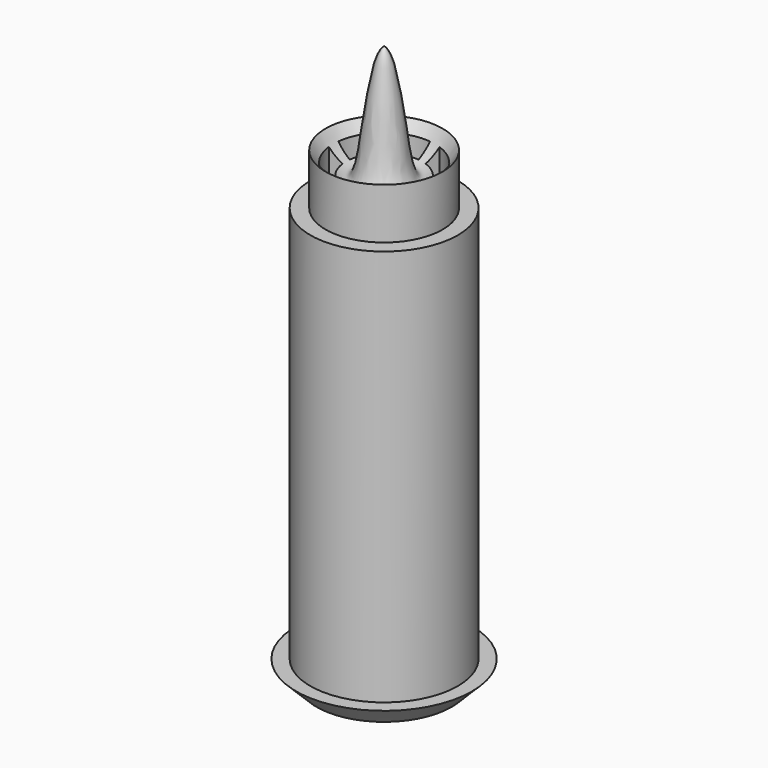
from build123d import *

# Parameters (mm, degrees)
F2_SIZE2  = 1.99999
F2_SIZE   = 1.99999
F5_R      = 5.75
F6_DEPTH  = 25
F7_R      = 5.75
F8_DEPTH  = 25
F10_DEPTH = 25


# Not quite as in the source:
# - a fillet or chamfer is up to 0.001 mm smaller than in the source, because OpenCascade refuses the exact size


with BuildPart() as f1:
    # F0 (on Front) → F1 (revolve)
    with BuildSketch(Plane.XZ):
        with BuildLine():
            Line((8.64674, 2), (7.25, 2))
            Line((7.25, 2), (7.25, 41))
            Line((7.25, 41), (5.75, 41))
            Line((5.75, 41), (5.75, 40))
            Line((5.75, 40), (4.75, 40))
            Line((4.75, 40), (4.75, 39))
            ThreePointArc((4.75, 39), (5.4571067812, 38.7071067812), (5.75, 38))
            Line((5.75, 38), (5.75, 4.9999998882))
            ThreePointArc((5.75, 4.9999998882), (5.4571067812, 4.2928931071), (4.75, 3.9999998882))
            Line((4.75, 3.9999998882), (4.75, 2.9999998882))
            Line((4.75, 2.9999998882), (5.75, 2.9999998882))
            Line((5.75, 2.9999998882), (5.75, 0))
            Line((5.75, 0), (8.64674, 0))
            Line((8.64674, 0), (8.64674, 2))
        make_face()
    revolve(axis=Axis((0, 0, 27.7979653329), (0, 0, 1)))

    # F2 (size 2 and 2 in the source; OpenCascade refuses exactly that, so slightly less here)
    f2_edges = [f1.edges().sort_by_distance(p)[0] for p in [
        (-8.64674, 0, 0),
    ]]
    chamfer(f2_edges, length=F2_SIZE, length2=F2_SIZE2)

    # F3 (on Front) → F4 (revolve)
    with BuildSketch(Plane.XZ):
        with BuildLine():
            Line((0, 55), (0, 41))
            Line((0, 41), (0, 40))
            Line((0, 40), (5.75, 40))
            Line((5.75, 40), (5.75, 46))
            add(Edge.make_bspline(
                [(0, 55), (0.1440579667, 54.8954034218), (0.4017096448, 54.5348723025), (0.9570213075, 53.3087861702), (1.7966593586, 47.7287211885), (2.1990543329, 44.2884011591), (2.9678127556, 43.2712194265), (4.3524509198, 44.1285353141), (5.1923480343, 45.0871969322), (5.5351351682, 45.7667505271), (5.75, 46)],
                knots=[0, 0, 0, 0, 0.0706016145, 0.1776436842, 0.4082606642, 0.5899939047, 0.6786962714, 0.7910306665, 0.9027344001, 1, 1, 1, 1], degree=3))
        make_face()
    revolve(axis=Axis((0, 0, 2), (0, 0, 1)))

    # F5 (on face) → F6 (cut)
    with BuildSketch(Plane(origin=(0, 0, 40), x_dir=(1, 0, 0), z_dir=(0, 0, -1))):
        Circle(F5_R)
    extrude(amount=F6_DEPTH, mode=Mode.SUBTRACT)

    # F7 (on face) → F8 (cut)
    with BuildSketch(Plane(origin=(0, 0, 2.9999998882), x_dir=(1, 0, 0), z_dir=(0, 0, -1))):
        Circle(F7_R)
    extrude(amount=-F8_DEPTH, mode=Mode.SUBTRACT)

    # F9 (on face) → F10 (cut)
    with BuildSketch(Plane(origin=(0, 0, 40), x_dir=(1, 0, 0), z_dir=(0, 0, -1))):
        with BuildLine():
            ThreePointArc((3.5453054724, 1.222010273), (3.75, 0), (3.5453054724, -1.222010273))
            Line((3.5453054724, -1.222010273), (4.7270739632, -1.6293470307))
            ThreePointArc((4.7270739632, -1.6293470307), (5, 0), (4.7270739632, 1.6293470307))
            Line((4.7270739632, 1.6293470307), (3.5453054724, 1.222010273))
        make_face()
        with BuildLine():
            Line((3.1658679099, 2.0099204903), (4.2211572131, 2.6798939871))
            ThreePointArc((4.2211572131, 2.6798939871), (3.1174490093, 3.9091574123), (1.6734076042, 4.7116565017))
            Line((1.6734076042, 4.7116565017), (1.2550557032, 3.5337423763))
            ThreePointArc((1.2550557032, 3.5337423763), (2.338086757, 2.9318680593), (3.1658679099, 2.0099204903))
        make_face()
        with BuildLine():
            Line((0.4024672392, 3.7283401295), (0.5366229857, 4.9711201727))
            ThreePointArc((0.5366229857, 4.9711201727), (-1.1126046698, 4.8746395609), (-2.640368812, 4.2459925267))
            Line((-2.640368812, 4.2459925267), (-1.980276609, 3.184494395))
            ThreePointArc((-1.980276609, 3.184494395), (-0.8344535023, 3.6559796707), (0.4024672392, 3.7283401295))
        make_face()
        with BuildLine():
            Line((-2.6639994714, 2.6392436069), (-3.5519992951, 3.5189914759))
            ThreePointArc((-3.5519992951, 3.5189914759), (-4.5048443395, 2.1694186956), (-4.9658936591, 0.5830095766))
            Line((-4.9658936591, 0.5830095766), (-3.7244202443, 0.4372571824))
            ThreePointArc((-3.7244202443, 0.4372571824), (-3.3786332546, 1.6270640217), (-2.6639994714, 2.6392436069))
        make_face()
        with BuildLine():
            Line((-3.7244202443, -0.4372571824), (-4.9658936591, -0.5830095766))
            ThreePointArc((-4.9658936591, -0.5830095766), (-4.5048443395, -2.1694186956), (-3.5519992951, -3.5189914759))
            Line((-3.5519992951, -3.5189914759), (-2.6639994714, -2.6392436069))
            ThreePointArc((-2.6639994714, -2.6392436069), (-3.3786332546, -1.6270640217), (-3.7244202443, -0.4372571824))
        make_face()
        with BuildLine():
            Line((-1.980276609, -3.184494395), (-2.640368812, -4.2459925267))
            ThreePointArc((-2.640368812, -4.2459925267), (-1.1126046698, -4.8746395609), (0.5366229857, -4.9711201727))
            Line((0.5366229857, -4.9711201727), (0.4024672392, -3.7283401295))
            ThreePointArc((0.4024672392, -3.7283401295), (-0.8344535023, -3.6559796707), (-1.980276609, -3.184494395))
        make_face()
        with BuildLine():
            Line((1.2550557032, -3.5337423763), (1.6734076042, -4.7116565017))
            ThreePointArc((1.6734076042, -4.7116565017), (3.1174490093, -3.9091574123), (4.2211572131, -2.6798939871))
            Line((4.2211572131, -2.6798939871), (3.1658679099, -2.0099204903))
            ThreePointArc((3.1658679099, -2.0099204903), (2.338086757, -2.9318680593), (1.2550557032, -3.5337423763))
        make_face()
    extrude(amount=-F10_DEPTH, mode=Mode.SUBTRACT)


solid = f1.part
